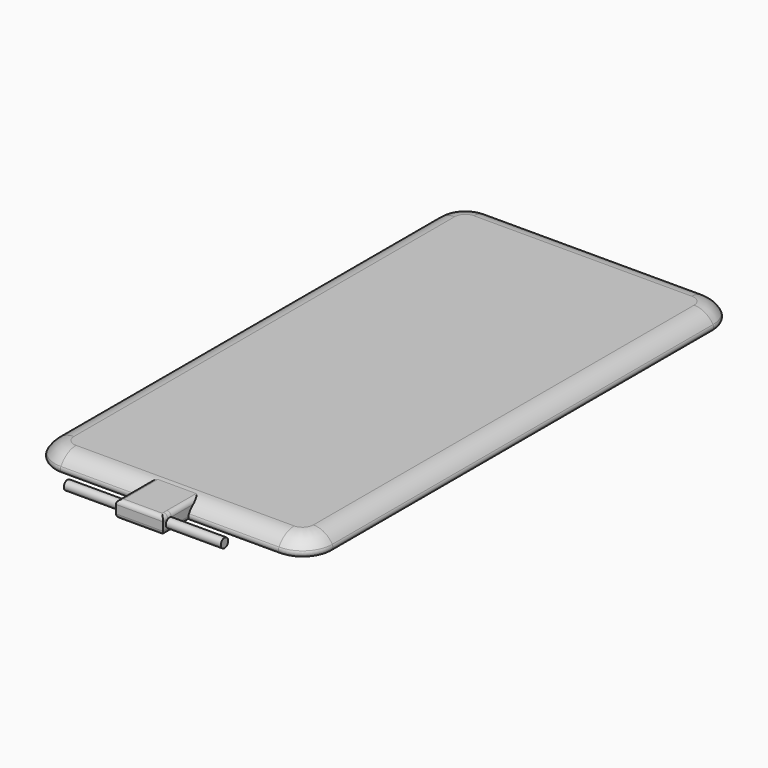
from build123d import *

# Parameters (mm, degrees)
F1_DEPTH     = 4
F2_T1_DEPTH  = 109.1
F2_T3_DEPTH  = 50
F2_T6_ANGLE  = 90
F2_T8_ANGLE  = 90
F2_T10_ANGLE = 90
F2_T12_ANGLE = 90
F3_R         = 1
F4_W         = 10.7876481488
F4_H         = 3.5392509308
F5_DEPTH     = 3.9
F6_DEPTH     = 4.8
F7_DEPTH     = 5
F8_R         = 1.0596630805
F9_DEPTH     = 18
F10_DEPTH    = 18
F11_R        = 1


# Not quite as in the source:
# - a fillet or chamfer that OpenCascade refuses, or shapes differently, is made with other operations: its cross-section is extruded or revolved along the edge and cut away or added


with BuildPart() as f1:
    # F0 (on Top) → F1 (new body)
    with BuildSketch(Plane.XY):
        with BuildLine():
            Line((26.0500038445, 123.900002712), (-23.9499961555, 123.900002712))
            ThreePointArc((-23.9499961555, 123.900002712), (-29.1472309972, 121.7472375537), (-31.2999961555, 116.550002712))
            Line((-31.2999961555, 116.550002712), (-31.2999961555, 7.450002712))
            ThreePointArc((-31.2999961555, 7.450002712), (-29.1472309972, 2.2527678703), (-23.9499961555, 0.100002712))
            Line((-23.9499961555, 0.100002712), (26.0500038445, 0.100002712))
            ThreePointArc((26.0500038445, 0.100002712), (31.2472386862, 2.2527678703), (33.4000038445, 7.450002712))
            Line((33.4000038445, 7.450002712), (33.4000038445, 116.550002712))
            ThreePointArc((33.4000038445, 116.550002712), (31.2472386862, 121.7472375537), (26.0500038445, 123.900002712))
        make_face()
    extrude(amount=F1_DEPTH)

    # F2: fillet of radius 5 on 1 edges, made by hand

    # F2_s2 → F2_t1 (cut)
    with BuildSketch(Plane.XZ.offset(-116.550002712)):
        with BuildLine():
            ThreePointArc((33.4000038445, 0), (31.6633020191, 2.8729833462), (28.5010243589, 4))
            Line((28.5010243589, 4), (28.5010243589, 4.1))
            Line((28.5010243589, 4.1), (33.4000038445, 4.1))
            Line((33.4000038445, 4.1), (33.5000038445, 4))
            ThreePointArc((33.5000038445, 4), (33.5000038445, 2), (33.4979834342, 0.02))
            Line((33.4979834342, 0.02), (33.4000038445, 0))
        make_face()
        with BuildLine():
            ThreePointArc((-31.2999961555, 0), (-29.5632943301, 2.8729833462), (-26.4010166699, 4))
            Line((-26.4010166699, 4), (-26.4010166699, 4.1))
            Line((-26.4010166699, 4.1), (-31.2999961555, 4.1))
            Line((-31.2999961555, 4.1), (-31.3999961555, 4))
            ThreePointArc((-31.3999961555, 4), (-31.3999961555, 2), (-31.3979757452, 0.02))
            Line((-31.3979757452, 0.02), (-31.2999961555, 0))
        make_face()
    extrude(amount=F2_T1_DEPTH, mode=Mode.SUBTRACT)

    # F2_s4 → F2_t3 (cut)
    with BuildSketch(Plane.YZ.offset(-23.9499961555)):
        with BuildLine():
            ThreePointArc((123.900002712, 0), (122.1633008866, 2.8729833462), (119.0010232264, 4))
            Line((119.0010232264, 4), (119.0010232264, 4.1))
            Line((119.0010232264, 4.1), (123.900002712, 4.1))
            Line((123.900002712, 4.1), (124.000002712, 4))
            ThreePointArc((124.000002712, 4), (124.000002712, 2), (123.9979823017, 0.02))
            Line((123.9979823017, 0.02), (123.900002712, 0))
        make_face()
        with BuildLine():
            ThreePointArc((0.100002712, 0), (1.8367045374, 2.8729833462), (4.9989821976, 4))
            Line((4.9989821976, 4), (4.9989821976, 4.1))
            Line((4.9989821976, 4.1), (0.100002712, 4.1))
            Line((0.100002712, 4.1), (2.712e-06, 4))
            ThreePointArc((2.712e-06, 4), (2.712e-06, 2), (0.0020231223, 0.02))
            Line((0.0020231223, 0.02), (0.100002712, 0))
        make_face()
    extrude(amount=F2_T3_DEPTH, mode=Mode.SUBTRACT)

    # F2_s5 → F2_t6 (revolve, cut)
    with BuildSketch(Plane.YZ.offset(26.0500038445)):
        with BuildLine():
            ThreePointArc((0.100002712, 0), (1.8367045374, 2.8729833462), (4.9989821976, 4))
            Line((4.9989821976, 4), (4.9989821976, 4.1))
            Line((4.9989821976, 4.1), (0.100002712, 4.1))
            Line((0.100002712, 4.1), (2.712e-06, 4))
            ThreePointArc((2.712e-06, 4), (2.712e-06, 2), (0.0020231223, 0.02))
            Line((0.0020231223, 0.02), (0.100002712, 0))
        make_face()
    revolve(axis=Axis((26.0500038445, 7.450002712, 4), (0, 0, 1)), revolution_arc=F2_T6_ANGLE, mode=Mode.SUBTRACT)

    # F2_s7 → F2_t8 (revolve, cut)
    with BuildSketch(Plane.XZ.offset(-116.550002712)):
        with BuildLine():
            ThreePointArc((33.4000038445, 0), (31.6633020191, 2.8729833462), (28.5010243589, 4))
            Line((28.5010243589, 4), (28.5010243589, 4.1))
            Line((28.5010243589, 4.1), (33.4000038445, 4.1))
            Line((33.4000038445, 4.1), (33.5000038445, 4))
            ThreePointArc((33.5000038445, 4), (33.5000038445, 2), (33.4979834342, 0.02))
            Line((33.4979834342, 0.02), (33.4000038445, 0))
        make_face()
    revolve(axis=Axis((26.0500038445, 116.550002712, 4), (0, 0, 1)), revolution_arc=F2_T8_ANGLE, mode=Mode.SUBTRACT)

    # F2_s9 → F2_t10 (revolve, cut)
    with BuildSketch(Plane.YZ.offset(-23.9499961555)):
        with BuildLine():
            ThreePointArc((123.900002712, 0), (122.1633008866, 2.8729833462), (119.0010232264, 4))
            Line((119.0010232264, 4), (119.0010232264, 4.1))
            Line((119.0010232264, 4.1), (123.900002712, 4.1))
            Line((123.900002712, 4.1), (124.000002712, 4))
            ThreePointArc((124.000002712, 4), (124.000002712, 2), (123.9979823017, 0.02))
            Line((123.9979823017, 0.02), (123.900002712, 0))
        make_face()
    revolve(axis=Axis((-23.9499961555, 116.550002712, 4), (0, 0, 1)), revolution_arc=F2_T10_ANGLE, mode=Mode.SUBTRACT)

    # F2_s11 → F2_t12 (revolve, cut)
    with BuildSketch(Plane.XZ.offset(-7.450002712)):
        with BuildLine():
            ThreePointArc((-31.2999961555, 0), (-29.5632943301, 2.8729833462), (-26.4010166699, 4))
            Line((-26.4010166699, 4), (-26.4010166699, 4.1))
            Line((-26.4010166699, 4.1), (-31.2999961555, 4.1))
            Line((-31.2999961555, 4.1), (-31.3999961555, 4))
            ThreePointArc((-31.3999961555, 4), (-31.3999961555, 2), (-31.3979757452, 0.02))
            Line((-31.3979757452, 0.02), (-31.2999961555, 0))
        make_face()
    revolve(axis=Axis((-23.9499961555, 7.450002712, 4), (0, 0, 1)), revolution_arc=F2_T12_ANGLE, mode=Mode.SUBTRACT)

    # F3
    f3_edges = [f1.edges().sort_by_distance(p)[0] for p in [
        (33.400004, 62.000003, 0),
        (31.247239, 121.747238, 0),
        (1.050004, 123.900003, 0),
        (-29.147231, 121.747238, 0),
        (-31.299996, 62.000003, 0),
        (-29.147231, 2.252768, 0),
        (1.050004, 0.100003, 0),
        (31.247239, 2.252768, 0),
    ]]
    fillet(f3_edges, radius=F3_R)

    # F4 (on Top) → F5 (join)
    with BuildSketch(Plane.XY):
        Rectangle(F4_W, F4_H)
    extrude(amount=F5_DEPTH)

    # F6 (add): a face of the model
    f6_faces = [f1.faces().sort_by_distance(p)[0] for p in [
        (0, 1.7696254654, 3.3586156696),
    ]]
    extrude(f6_faces, amount=F6_DEPTH)

    # F7 (add): a face of the model
    f7_faces = [f1.faces().sort_by_distance(p)[0] for p in [
        (0, -1.7696254654, 1.95),
    ]]
    extrude(f7_faces, amount=F7_DEPTH)

    # F8 (on Right) → F9 (join)
    with BuildSketch(Plane.YZ):
        with Locations((-4.8954286613, 1.9693823997)):
            Circle(F8_R)
    extrude(amount=F9_DEPTH)

    # F8 (on Right) → F10 (join)
    with BuildSketch(Plane.YZ):
        with Locations((-4.8954286613, 1.9693823997)):
            Circle(F8_R)
    extrude(amount=-F10_DEPTH)

    # F11
    f11_edges = [f1.edges().sort_by_distance(p)[0] for p in [
        (5.393824, -1.382815, 3.9),
        (-5.393824, -1.382815, 3.9),
        (0, -6.769625, 3.9),
        (0, -6.769625, 0),
        (5.393824, -2.617372, 0),
        (-5.393824, -2.617372, 0),
    ]]
    fillet(f11_edges, radius=F11_R)


solid = f1.part
